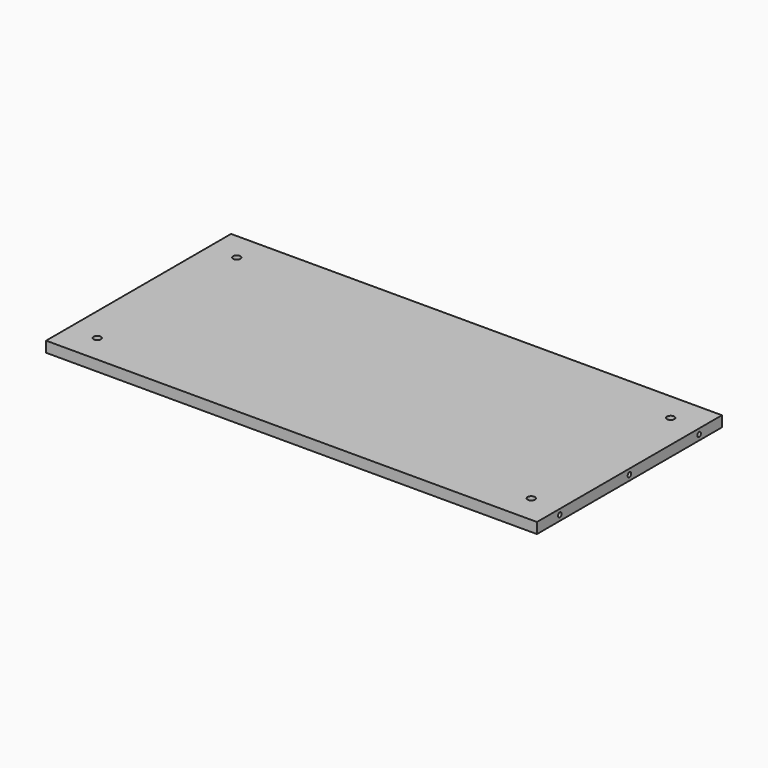
from build123d import *

# Parameters (mm, degrees)
F0_W      = 876.3
F0_H      = 412.75
F1_DEPTH  = 19.05
F3_D      = 15.0114
F3_DEPTH  = 14.224
F3_TIP    = 4.5098795482
F5_D      = 8.001
F5_DEPTH  = 25.4
F5_TIP    = 2.4037429064
F7_D      = 8.001
F7_DEPTH  = 25.4
F7_TIP    = 2.4037429064
F9_D      = 8.001
F9_DEPTH  = 25.4
F9_TIP    = 2.4037429064
F11_D     = 12.9794
F11_DEPTH = 25.4
F11_TIP   = 3.8994051593


with BuildPart() as f1:
    # F0 (on Top) → F1 (new body)
    with BuildSketch(Plane.XY):
        Rectangle(F0_W, F0_H)
    extrude(amount=F1_DEPTH)

    # F3
    with Locations(Plane(origin=(0, 0, 0), x_dir=(1, 0, 0), z_dir=(0, 0, -1))):
        with Locations((-414.274, 155.575), (-414.274, 0), (-414.274, -155.575), (-387.35, -182.499), (0, -182.499), (387.35, -182.499), (414.274, -155.575), (414.274, 0), (414.274, 155.575)):
            Hole(F3_D / 2, depth=F3_DEPTH)
            with Locations((0, 0, -(F3_DEPTH + F3_TIP / 2))):  # 118° drill point
                Cone(0, F3_D / 2, F3_TIP, mode=Mode.SUBTRACT)

    # F5
    with Locations(Plane(origin=(0, 206.375, 0), x_dir=(-1, 0, 0), z_dir=(0, 1, 0))):
        with Locations((-387.35, 9.525), (0, 9.525), (387.35, 9.525)):
            Hole(F5_D / 2, depth=F5_DEPTH)
            with Locations((0, 0, -(F5_DEPTH + F5_TIP / 2))):  # 118° drill point
                Cone(0, F5_D / 2, F5_TIP, mode=Mode.SUBTRACT)

    # F7
    with Locations(Plane(origin=(-438.15, 0, 0), x_dir=(0, -1, 0), z_dir=(-1, 0, 0))):
        with Locations((-155.575, 9.525), (0, 9.525), (155.575, 9.525)):
            Hole(F7_D / 2, depth=F7_DEPTH)
            with Locations((0, 0, -(F7_DEPTH + F7_TIP / 2))):  # 118° drill point
                Cone(0, F7_D / 2, F7_TIP, mode=Mode.SUBTRACT)

    # F9
    with Locations(Plane.YZ.offset(438.15)):
        with Locations((-155.575, 9.525), (0, 9.525), (155.575, 9.525)):
            Hole(F9_D / 2, depth=F9_DEPTH)
            with Locations((0, 0, -(F9_DEPTH + F9_TIP / 2))):  # 118° drill point
                Cone(0, F9_D / 2, F9_TIP, mode=Mode.SUBTRACT)

    # F11
    with Locations(Plane.XY.offset(19.05)):
        with Locations((-387.35, 155.575), (387.35, 155.575), (387.35, -155.575), (-387.35, -155.575)):
            Hole(F11_D / 2, depth=F11_DEPTH)
            with Locations((0, 0, -(F11_DEPTH + F11_TIP / 2))):  # 118° drill point
                Cone(0, F11_D / 2, F11_TIP, mode=Mode.SUBTRACT)


solid = f1.part
